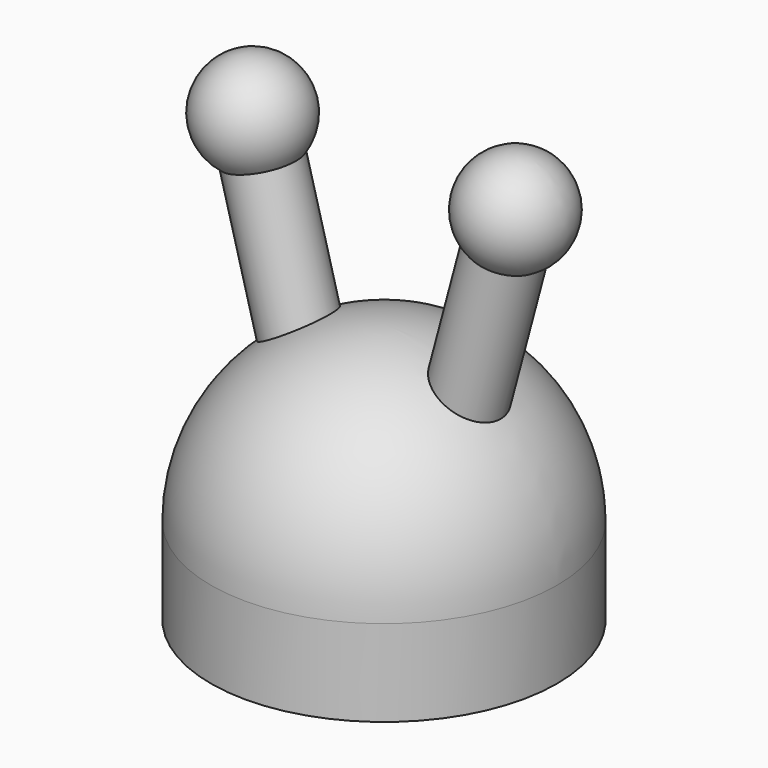
from build123d import *


# Not quite as in the source:
# - a pattern or mirror of a feature is missing from the dataset's text; its kind, count and spacing are read off the source's solid


with BuildPart() as f1:
    # F0 (on Front) → F1 (revolve)
    with BuildSketch(Plane.XZ):
        with BuildLine():
            ThreePointArc((0, 25), (2.5, 24.3301270189), (4.3301270189, 22.5))
            Line((4.3301270189, 22.5), (17.3205080757, 0))
            Line((17.3205080757, 0), (20, 0))
            Line((20, 0), (20, 10))
            ThreePointArc((20, 10), (14.1421356237, 24.1421356237), (0, 30))
            Line((0, 30), (0, 25))
        make_face()
    revolve(axis=Axis((0, 0, 15), (0, 0, 1)))

    # F2 (on Front) → F3 (revolve)
    with BuildSketch(Plane.XZ):
        with BuildLine():
            Line((15.1763809021, 46.6390246015), (9.3060056246, 24.7304858066))
            Line((9.3060056246, 24.7304858066), (13.1697089298, 23.6952096262))
            Line((13.1697089298, 23.6952096262), (17.8826102498, 41.2839968035))
            ThreePointArc((17.8826102498, 41.2839968035), (21.1445422637, 47.2563170454), (16.7292951727, 52.4345795592))
            Line((16.7292951727, 52.4345795592), (15.1763809021, 46.6390246015))
        make_face()
    f3 = revolve(axis=Axis((12.2411932633, 0, 35.684755204), (-0.2588190451, 0, -0.9659258263)))

    # F3_copies: F3 across plane
    add(f3.mirror(Plane(origin=(-2.2e-05, 0, 0), x_dir=(0, 0, -1), z_dir=(-1, 0, 0))))


solid = f1.part
